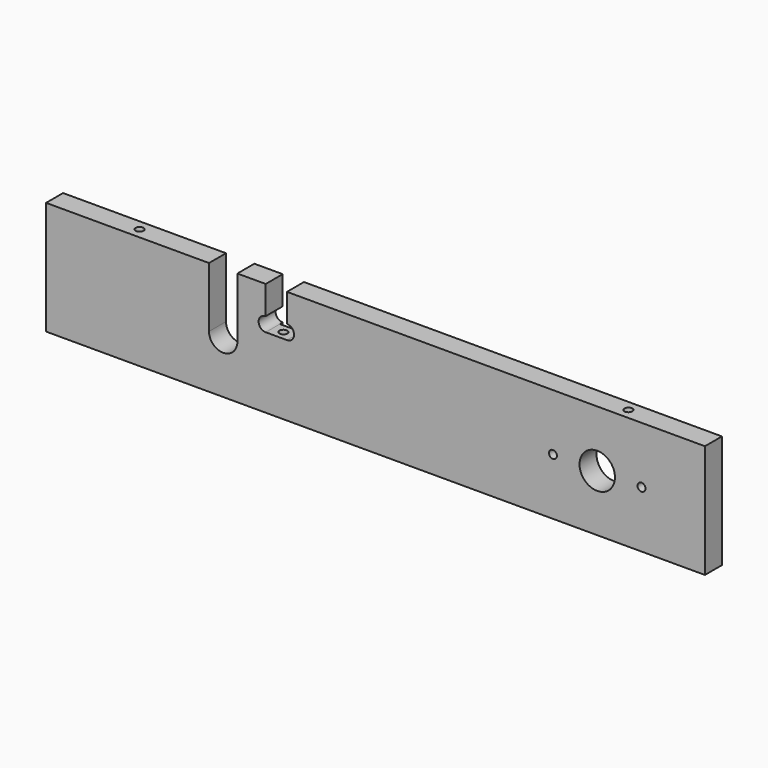
from build123d import *

# Parameters (mm, degrees)
F0_R             = 1.7859375
F0_R_2           = 7.9375
F1_DEPTH         = 9.525
F2_W             = 9.5377
F2_H             = 31.75
F3_DEPTH         = 1.5875
F5_D             = 3.571875
F5_DEPTH         = 19.05
F5_TIP           = 1.0730995118
F7_D             = 3.571875
F7_DEPTH         = 19.05
F7_TIP           = 1.0730995118
F11_D            = 3.571875
F11_DEPTH        = 12.7
F11_TIP          = 1.0730995118
F11_ON_F9_D      = 3.571875
F11_ON_F9_DEPTH  = 12.7
F11_ON_F9_TIP    = 1.0730995118
F11_ON_F10_D     = 3.571875
F11_ON_F10_DEPTH = 12.7
F11_ON_F10_TIP   = 1.0730995118


# Not quite as in the source:
# - a feature names something its author has since deleted; it is built from what else it names


with BuildPart() as f1:
    # F0 (on Front) → F1 (new body)
    with BuildSketch(Plane.XZ):
        with BuildLine():
            Line((0, 50.8), (0, 0))
            Line((0, 0), (295.275, 0))
            Line((295.275, 0), (295.275, 50.8))
            Line((295.275, 50.8), (107.9627, 50.8))
            Line((107.9627, 50.8), (107.9627, 38.1))
            ThreePointArc((107.9627, 38.1), (111.1377, 34.925), (107.9627, 31.75))
            Line((107.9627, 31.75), (98.425, 31.75))
            ThreePointArc((98.425, 31.75), (95.25, 34.925), (98.425, 38.1))
            Line((98.425, 38.1), (98.425, 50.8))
            Line((98.425, 50.8), (85.725, 50.8))
            Line((85.725, 50.8), (85.725, 23.8125))
            ThreePointArc((85.725, 23.8125), (79.375, 17.4625), (73.025, 23.8125))
            Line((73.025, 23.8125), (73.025, 50.8))
            Line((73.025, 50.8), (0, 50.8))
        make_face()
        with Locations((227.17125, 25.4)):
            Circle(F0_R, mode=Mode.SUBTRACT)
        with Locations((247.015, 25.4)):
            Circle(F0_R_2, mode=Mode.SUBTRACT)
        with Locations((266.85875, 25.4)):
            Circle(F0_R, mode=Mode.SUBTRACT)
    extrude(amount=F1_DEPTH)

    # F2 (on face) → F3 (cut)
    with BuildSketch(Plane(origin=(0, 0, 0), x_dir=(-1, 0, 0), z_dir=(0, 1, 0))):
        with Locations((-103.19385, 15.875)):
            Rectangle(F2_W, F2_H)
    extrude(amount=-F3_DEPTH, mode=Mode.SUBTRACT)

    # F5
    with Locations(Plane(origin=(0, 0, 0), x_dir=(0, -1, 0), z_dir=(-1, 0, 0))):
        with Locations((4.7625, 38.1), (4.7625, 25.4), (4.7625, 12.7)):
            Hole(F5_D / 2, depth=F5_DEPTH)
            with Locations((0, 0, -(F5_DEPTH + F5_TIP / 2))):  # 118° drill point
                Cone(0, F5_D / 2, F5_TIP, mode=Mode.SUBTRACT)

    # F7
    with Locations(Plane.XY.offset(31.75)):
        with Locations((103.19385, -5.55625)):
            Hole(F7_D / 2, depth=F7_DEPTH)
            with Locations((0, 0, -(F7_DEPTH + F7_TIP / 2))):  # 118° drill point
                Cone(0, F7_D / 2, F7_TIP, mode=Mode.SUBTRACT)

    # F11
    with Locations(Plane.XY.offset(50.8)):
        with Locations((257.175, -4.7625)):
            Hole(F11_D / 2, depth=F11_DEPTH)
            with Locations((0, 0, -(F11_DEPTH + F11_TIP / 2))):  # 118° drill point
                Cone(0, F11_D / 2, F11_TIP, mode=Mode.SUBTRACT)

    # F11 on F9
    with Locations(Plane.XY.offset(50.8)):
        with Locations((38.1, -4.7625)):
            Hole(F11_ON_F9_D / 2, depth=F11_ON_F9_DEPTH)
            with Locations((0, 0, -(F11_ON_F9_DEPTH + F11_ON_F9_TIP / 2))):  # 118° drill point
                Cone(0, F11_ON_F9_D / 2, F11_ON_F9_TIP, mode=Mode.SUBTRACT)

    # F11 on F10
    with Locations(Plane(origin=(0, 0, 0), x_dir=(1, 0, 0), z_dir=(0, 0, -1))):
        with Locations((38.1, 4.7625), (257.175, 4.7625)):
            Hole(F11_ON_F10_D / 2, depth=F11_ON_F10_DEPTH)
            with Locations((0, 0, -(F11_ON_F10_DEPTH + F11_ON_F10_TIP / 2))):  # 118° drill point
                Cone(0, F11_ON_F10_D / 2, F11_ON_F10_TIP, mode=Mode.SUBTRACT)


solid = f1.part
